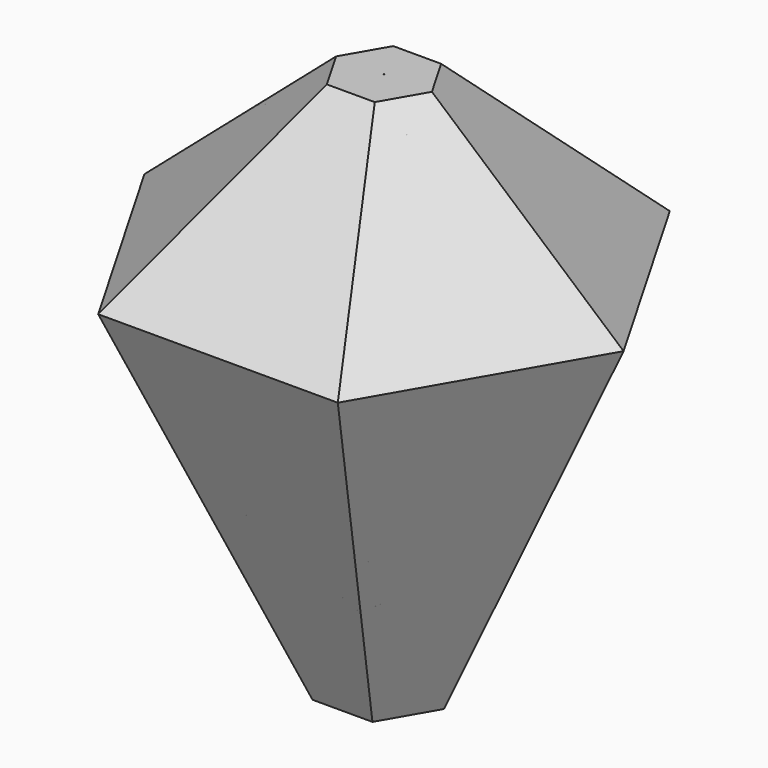
from build123d import *

# Parameters (mm, degrees)
F8_R      = 1
F9_DEPTH  = 5
F14_COUNT = 6


# Not quite as in the source:
# - a feature names something its author has since deleted; it is built from what else it names


with BuildPart() as f6:
    # F1 (on Top) → F6 section 0
    with BuildSketch(Plane.XY):
        Polygon((288.6751345948, 500), (-288.6751345948, 500), (-577.3502691896, 0), (-288.6751345948, -500), (288.6751345948, -500), (577.3502691896, 0), align=None)
    # F3 (on offset) → F6 section 1
    with BuildSketch(Plane.XY.offset(400)):
        Polygon((57.735026919, 100), (-57.735026919, 100), (-115.4700538379, 0), (-57.735026919, -100), (57.735026919, -100), (115.4700538379, 0), align=None)
    loft()

    # F5 (on offset) → F7 section 0
    with BuildSketch(Plane.XY.offset(-900)):
        Polygon((-72.1687836487, -125), (72.1687836487, -125), (144.3375672974, 0), (72.1687836487, 125), (-72.1687836487, 125), (-144.3375672974, 0), align=None)
    # F6_face (on face) → F7 section 1
    with BuildSketch(Plane(origin=(0, 0, 0), x_dir=(1, 0, 0), z_dir=(0, 0, -1))):
        Polygon((288.6751345948, -500), (577.3502691896, 0), (288.6751345948, 500), (-288.6751345948, 500), (-577.3502691896, 0), (-288.6751345948, -500), align=None)
    loft()

    # F8 (on face) → F9 (cut)
    with BuildSketch(Plane.XY.offset(400)):
        Circle(F8_R)
    extrude(amount=-F9_DEPTH, mode=Mode.SUBTRACT)


with BuildPart() as f14_1:
    # F14: instance of F6
    add(f6.part.rotate(Axis((0, 0, 3.9595463313), (0, 0, 1)), 1 * 360 / F14_COUNT))


with BuildPart() as f14_2:
    # F14: instance of F6
    add(f6.part.rotate(Axis((0, 0, 3.9595463313), (0, 0, 1)), 2 * 360 / F14_COUNT))


with BuildPart() as f14_3:
    # F14: instance of F6
    add(f6.part.rotate(Axis((0, 0, 3.9595463313), (0, 0, 1)), 3 * 360 / F14_COUNT))


with BuildPart() as f14_4:
    # F14: instance of F6
    add(f6.part.rotate(Axis((0, 0, 3.9595463313), (0, 0, 1)), 4 * 360 / F14_COUNT))


with BuildPart() as f14_5:
    # F14: instance of F6
    add(f6.part.rotate(Axis((0, 0, 3.9595463313), (0, 0, 1)), 5 * 360 / F14_COUNT))


solid = Compound([f6.part, f14_1.part, f14_2.part, f14_3.part, f14_4.part, f14_5.part])
